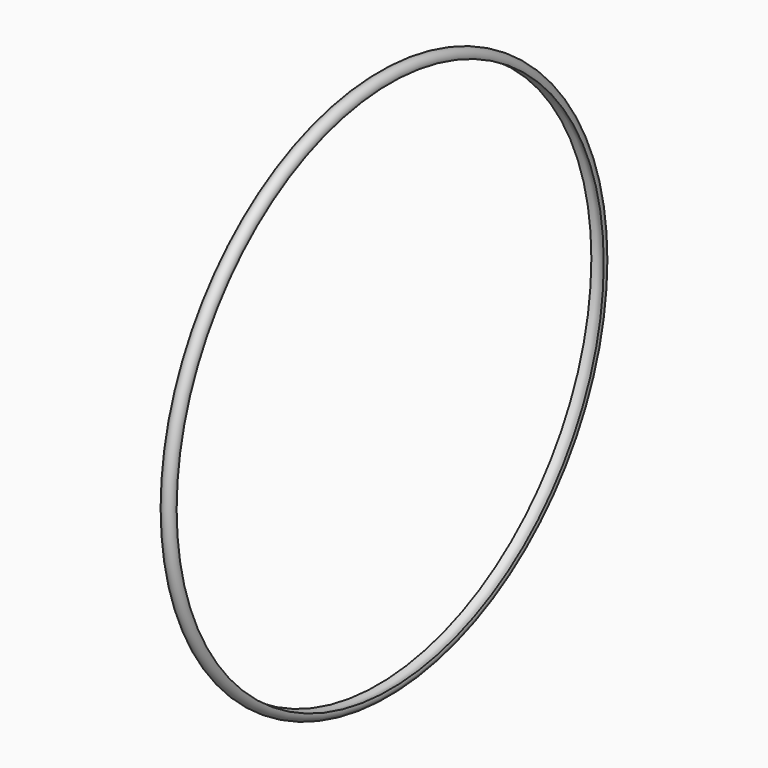
from build123d import *


# Not quite as in the source:
# - a feature names something its author has since deleted; it is built from what else it names
# - the program builds the solid bodies; features that only make, move or delete a surface that nothing else refers to are left out


with BuildPart() as f3:
    # F3: sweep along a path in F0
    with BuildLine(Plane.YZ) as f3_path:
        CenterArc((-44.45, -25.4), 19.05, 0, 360)
    # F2 (on offset) → F3 (sweep)
    with BuildSketch(Plane.XZ.offset(44.45)):
        with BuildLine():
            add(Edge.make_bspline(
                [(-0.4318, -6.7860578887), (-0.2878666667, -6.7190095517), (0, -6.5849128778), (0.2878666667, -6.7190095517), (0.4318, -6.7860578887)],
                knots=[0, 0, 0, 0, 0.5, 1, 1, 1, 1], degree=3))
            ThreePointArc((0.4318, -6.7860578887), (0, -6.1998183635), (-0.4318, -6.7860578887))
        make_face()
    sweep(path=f3_path.line)


solid = f3.part
